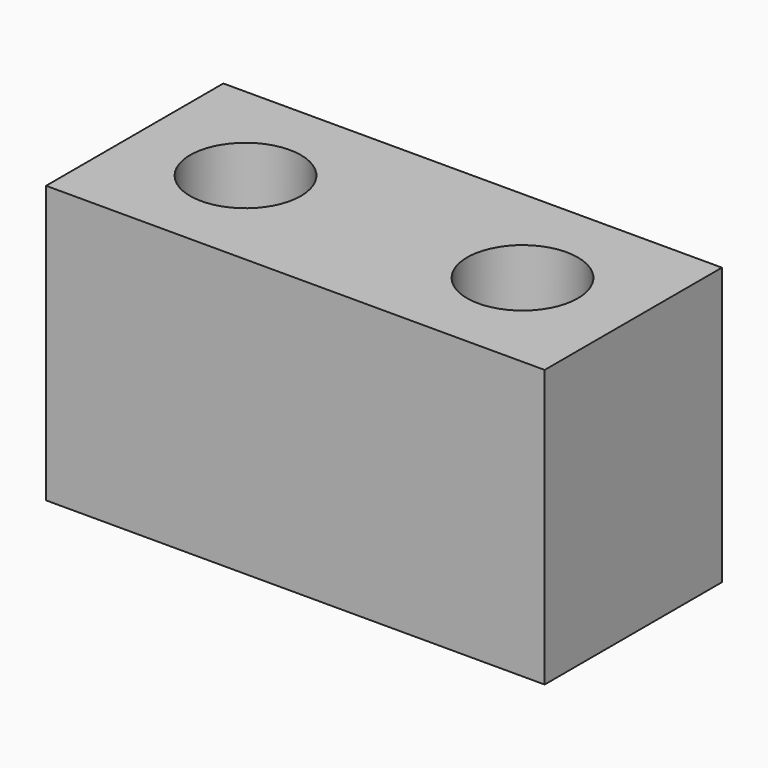
from build123d import *

# Parameters (mm, degrees)
F0_W     = 9
F0_H     = 4
F0_R     = 1
F1_DEPTH = 5


# Not quite as in the source:
# - the program builds the solid bodies; features that only make, move or delete a surface that nothing else refers to are left out


with BuildPart() as f1:
    # F0 (on Top) → F1 (new body)
    with BuildSketch(Plane.XY):
        Rectangle(F0_W, F0_H)
        with Locations((-2.5, 0)):
            Circle(F0_R, mode=Mode.SUBTRACT)
        with Locations((2.5, 0)):
            Circle(F0_R, mode=Mode.SUBTRACT)
    extrude(amount=F1_DEPTH)


solid = f1.part
